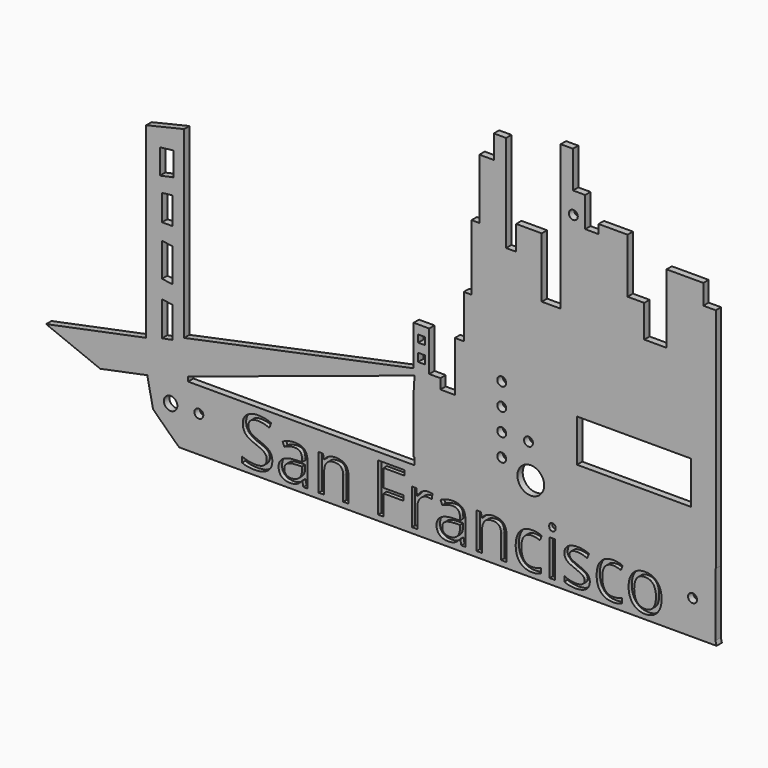
from build123d import *

# Parameters (mm, degrees)
F0_W         = 2.9822538366
F0_H         = 3.6448612809
F0_W_2       = 135.3491628077
F0_H_2       = 25.4928320646
F1_DEPTH     = 3
F3_W         = 51.13
F3_H         = 19.04
F3_R         = 2
F3_R_2       = 6
F3_R_3       = 3
F4_DEPTH     = 53
F5_DEPTH     = 3
F6_TEXT_SIZE = 30.0559525688
F7_DEPTH     = 8.3
F8_DEPTH     = 1.2
F9_R         = 2
F10_DEPTH    = 36
F11_DEPTH    = 80


# Not quite as in the source:
# - Text() gives the source's letters only with a copy of the font that has no kerning and outlines rounded to 1/6400 em; it was checked with that copy


with BuildPart() as f1:
    # F0 (on Front) → F1 (new body)
    with BuildSketch(Plane.XZ):
        Polygon((47.3068803549, -141.5077000856), (2.4387890007, -150.6752371788), (26.6882968148, -160.4099207076), (47.7795305522, -156.1005181502), (50.3422312246, -168.6429803961), (60.1621009409, -178.1576573849), (66.0483464599, -178.1576573849), (66.0483464599, -150.6752371788), (167.5079911947, -117.3093244433), (167.089626193, -124.0393817425), (302.4387890007, -124.0393817425), (302.4387890007, -47.6778820157), (296.8542873859, -47.6778820157), (296.8542873859, -38.6941768229), (280.3841531277, -38.6941768229), (280.3841531277, -69.6380510926), (270.4022526741, -69.6380510926), (270.4022526741, -55.1643036306), (262.9158198833, -55.1643036306), (262.9158198833, -30.7086613029), (249.9393671751, -30.7086613029), (249.9393671751, -34.7014181316), (243.9502328634, -34.7014181316), (243.9502328634, -21.2258584797), (238.4601831436, -21.2258584797), (238.4601831436, -4.7557349317), (232.970148325, -4.7557349317), (232.970148325, -69.6380510926), (224.4855314493, -69.6380510926), (224.4855314493, -42.6869355142), (213.0063474178, -42.6869355142), (213.0063474178, -53.6670200527), (208.5144966841, -53.6670200527), (208.5144966841, -10.2457767352), (203.0244469643, -10.2457767352), (203.0244469643, -20.7267645746), (196.5362280607, -20.7267645746), (196.5362280607, -47.6778820157), (193.0425614119, -47.6778820157), (193.0425614119, -77.1244764328), (189.548894763, -77.1244764328), (189.548894763, -96.5891703963), (185.5561286211, -96.5891703963), (185.5561286211, -119.0484389663), (179.0678948164, -119.0484389663), (179.0678948164, -114.5565807819), (174.0769594908, -114.5565807819), (174.0769594908, -96.5891703963), (167.089626193, -96.5891703963), (167.089626193, -114.5565807819), (64.2761066556, -136.0176503658), (64.2761066556, -53.6670200527), (47.3068803549, -57.659778744), align=None)
        Polygon((54.393991828, -139.3551230431), (54.393991828, -123.9771693945), (59.1402724385, -124.641649425), (59.1402724385, -138.5007798672), align=None, mode=Mode.SUBTRACT)
        Polygon((59.1402724385, -116.5729686618), (54.393991828, -115.9084886312), (54.393991828, -100.9102389216), (59.1402724385, -101.5747189522), align=None, mode=Mode.SUBTRACT)
        with Locations((170.592171454, -109.5926128328)):
            Rectangle(F0_W, F0_H, mode=Mode.SUBTRACT)
        Polygon((169.1010445356, -103.7939712405), (169.1010445356, -100.5633026361), (172.0832983723, -100.5633026361), (172.0832983723, -103.7971321213), align=None, mode=Mode.SUBTRACT)
        Polygon((54.393991828, -82.0208713412), (59.1402724385, -81.4810320735), (59.1402724385, -93.6272367835), (54.393991828, -93.6272367835), align=None, mode=Mode.SUBTRACT)
        Polygon((53.4260459244, -75.5300670862), (53.4260459244, -64.3651112914), (59.6287995577, -63.6207833886), (59.6287995577, -74.227489531), align=None, mode=Mode.SUBTRACT)
        with Locations((234.7642075969, -136.7857977748)):
            Rectangle(F0_W_2, F0_H_2)
    extrude(amount=F1_DEPTH)

    # F3 (on Front) → F4 (cut)
    with BuildSketch(Plane.XZ):
        with Locations((265.8203148985, -119.2788640986)):
            Rectangle(F3_W, F3_H)
        with Locations((206.5561286211, -116.9127482176)):
            Circle(F3_R)
        with Locations((206.5561286211, -126.9127482176)):
            Circle(F3_R)
        with Locations((218.5561286211, -126.7215162516)):
            Circle(F3_R)
        with Locations((206.5561286211, -136.9127482176)):
            Circle(F3_R)
        with Locations((206.5561286211, -106.9127482176)):
            Circle(F3_R)
        with Locations((219.5561286211, -141.7215162516)):
            Circle(F3_R_2)
        with Locations((58.2325134349, -163.7986080633)):
            Circle(F3_R_3)
    extrude(amount=F4_DEPTH, mode=Mode.SUBTRACT)

    # F2 (on Front) → F5 (join)
    with BuildSketch(Plane.XZ):
        Polygon((302.2848069668, -178.0121773481), (302.2848069668, -124.3897154927), (302.2478222847, -123.8509938121), (296.3267791347, -123.8509938121), (296.3267791347, -149.1422504187), (296.3267791347, -150.9315855801), (296.3267791347, -152.6724770665), (296.3267791347, -178.0121773481), align=None)
        Polygon((302.7981519699, -179.8944920301), (302.2848069668, -178.0121773481), (296.3267791347, -178.0121773481), (72.2233057022, -178.0121773481), (65.715149045, -178.0121773481), (60.1672455668, -178.147688508), (62.0935633779, -179.8944920301), align=None)
        Polygon((72.2233057022, -178.0121773481), (296.3267791347, -178.0121773481), (296.3267791347, -152.6724770665), (173.9494204521, -152.6724770665), (167.5813496113, -152.6724770665), (72.2233057022, -152.6724770665), align=None)
        Polygon((65.715149045, -178.0121773481), (72.2233057022, -178.0121773481), (72.2233057022, -152.6724770665), (66.1221593618, -152.6724770665), (65.9683405805, -162.2489463963), align=None)
        Polygon((173.9494204521, -152.6724770665), (296.3267791347, -152.6724770665), (296.3267791347, -150.9315855801), (173.9494204521, -149.2145955563), align=None)
        Polygon((296.3267791347, -150.9315855801), (296.3267791347, -149.1422504187), (296.0256934166, -149.1422504187), (173.9494204521, -149.2145955563), align=None)
        Polygon((167.5813496113, -152.6724770665), (173.9494204521, -152.6724770665), (173.9494204521, -149.2145955563), (173.9494204521, -124.465033412), (173.9494204521, -124.0292191505), (167.5813496113, -124.0292191505), (167.5813496113, -124.0914985538), (167.5813496113, -124.465033412), align=None)
        Polygon((65.8576662108, -152.6682287352), (65.9683405805, -162.2489463963), (66.1221593618, -152.6724770665), align=None)
    extrude(amount=F5_DEPTH)

    # F6 (on Front) → F7 (cut)
    with BuildSketch(Plane.XZ):
        with Locations((88.7291580439, -177.474245429)):
            Text('San Francisco', F6_TEXT_SIZE, font='Open Sans', text_align=(TextAlign.LEFT, TextAlign.BOTTOM))
    extrude(amount=F7_DEPTH, mode=Mode.SUBTRACT)

    # F9 (on Front) → F10 (cut)
    with BuildSketch(Plane.XZ):
        with Locations((238.6275231838, -30.8220889419)):
            Circle(F9_R)
        with Locations((292.0418679714, -164.5557880402)):
            Circle(F9_R)
        with Locations((70.8668977022, -163.764461875)):
            Circle(F9_R)
    extrude(amount=F10_DEPTH, mode=Mode.SUBTRACT)

    # F3 (on Front) → F11 (cut)
    with BuildSketch(Plane.XZ):
        with Locations((265.8203148985, -119.2788640986)):
            Rectangle(F3_W, F3_H)
        with Locations((206.5561286211, -116.9127482176)):
            Circle(F3_R)
        with Locations((206.5561286211, -126.9127482176)):
            Circle(F3_R)
        with Locations((218.5561286211, -126.7215162516)):
            Circle(F3_R)
        with Locations((206.5561286211, -136.9127482176)):
            Circle(F3_R)
        with Locations((206.5561286211, -106.9127482176)):
            Circle(F3_R)
        with Locations((219.5561286211, -141.7215162516)):
            Circle(F3_R_2)
        with Locations((58.2325134349, -163.7986080633)):
            Circle(F3_R_3)
    extrude(amount=-F11_DEPTH, mode=Mode.SUBTRACT)


with BuildPart() as f8:
    # F6 (on Front) → F8 (new body)
    with BuildSketch(Plane.XZ):
        with Locations((88.7291580439, -177.474245429)):
            Text('San Francisco', F6_TEXT_SIZE, font='Open Sans', text_align=(TextAlign.LEFT, TextAlign.BOTTOM))
    extrude(amount=F8_DEPTH)


solid = Compound([f1.part, f8.part])
